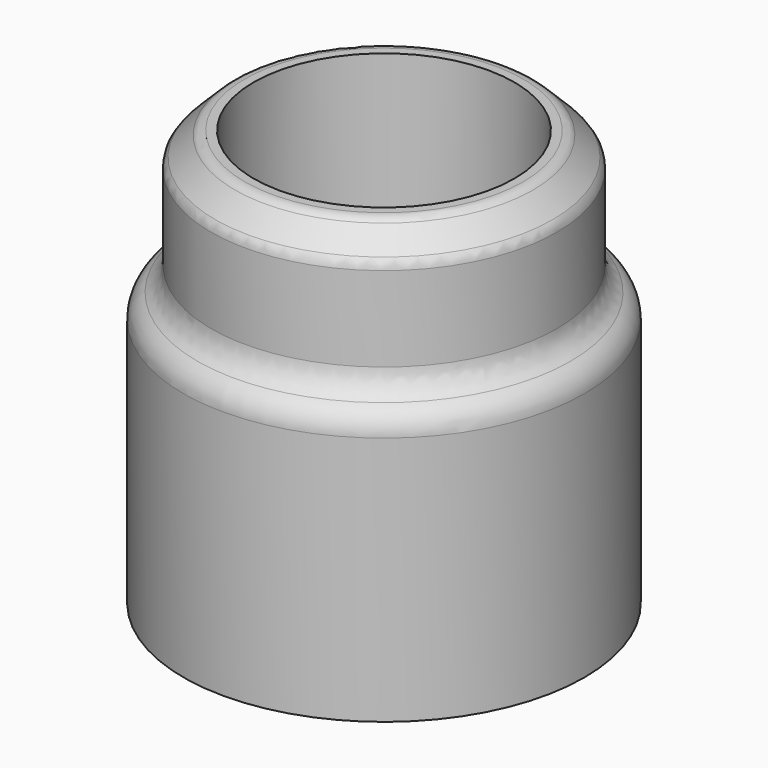
from build123d import *

# Parameters (mm, degrees)
F0_R     = 36.6966973779
F1_DEPTH = 50.8
F2_R     = 5.08
F3_R     = 23.8679289638
F4_DEPTH = 13.208
F5_DEPTH = 25.4
F6_R     = 5.08
F7_SIZE  = 5.08
F8_R     = 2.54


# Not quite as in the source:
# - two fillets or chamfers of one size are made in one step


with BuildPart() as f1:
    # F0 (on Top) → F1 (new body)
    with BuildSketch(Plane.XY):
        Circle(F0_R)
    extrude(amount=F1_DEPTH)

    # F2
    f2_edges = [f1.edges().sort_by_distance(p)[0] for p in [
        (-36.696697, 0, 50.8),
    ]]
    fillet(f2_edges, radius=F2_R)

    # F3 (on face) → F4 (cut)
    with BuildSketch(Plane.XY.offset(50.8)):
        Circle(F3_R)
    extrude(amount=-F4_DEPTH, mode=Mode.SUBTRACT)

    # F5 (add): a face of the model
    f5_faces = [f1.faces().sort_by_distance(p)[0] for p in [
        (-30.7224421333, 0, 50.8),
    ]]
    extrude(f5_faces, amount=F5_DEPTH)

    # F6
    f6_edges = [f1.edges().sort_by_distance(p)[0] for p in [
        (-31.616697, 0, 50.8),
    ]]
    fillet(f6_edges, radius=F6_R)

    # F7
    f7_edges = [f1.edges().sort_by_distance(p)[0] for p in [
        (-31.616697, 0, 76.2),
    ]]
    chamfer(f7_edges, length=F7_SIZE)

    # F8
    f8_edges = [f1.edges().sort_by_distance(p)[0] for p in [
        (-31.616697, 0, 71.12),
        (-26.536697, 0, 76.2),
    ]]
    fillet(f8_edges, radius=F8_R)


solid = f1.part
